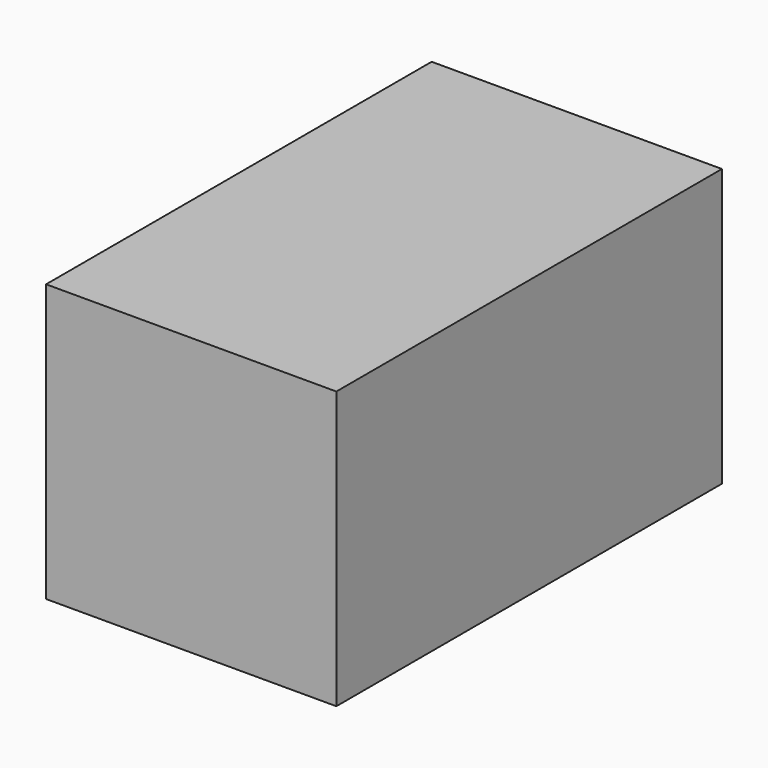
from build123d import *

# Parameters (mm, degrees)
F0_W     = 60.2300651371
F0_H     = 57.4923343956
F1_DEPTH = 100


# Not quite as in the source:
# - the program builds the solid bodies; features that only make, move or delete a surface that nothing else refers to are left out


with BuildPart() as f1:
    # F0 (on Front) → F1 (new body)
    with BuildSketch(Plane.XZ):
        with Locations((30.1150325686, 28.7461671978)):
            Rectangle(F0_W, F0_H)
    extrude(amount=F1_DEPTH)


solid = f1.part
